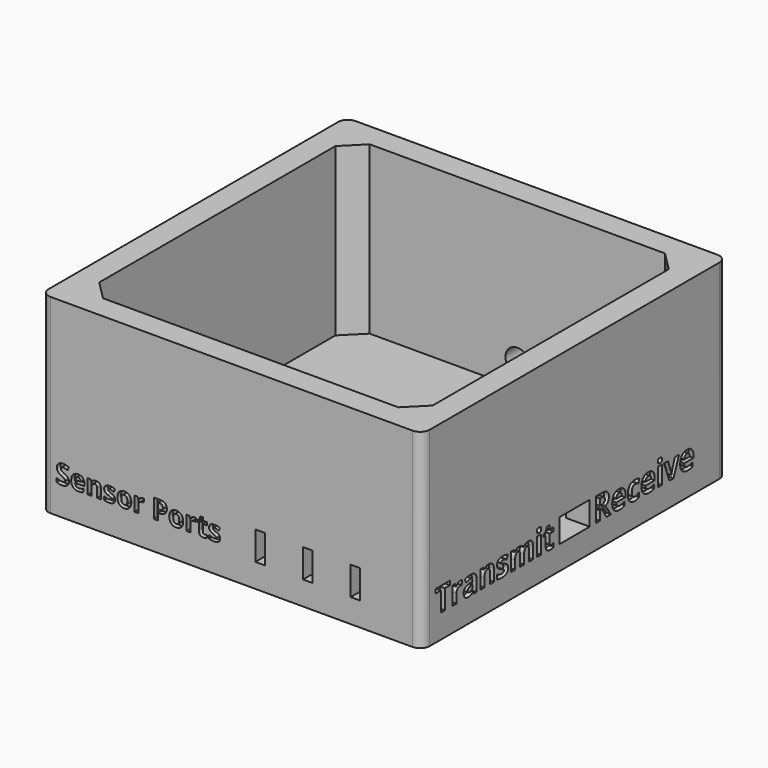
from build123d import *

# Parameters (mm, degrees)
F0_W          = 101.6
F0_H          = 101.6
F1_DEPTH      = 50.8
F2_T          = -6.35
F3_TEXT_SIZE  = 8.8194444444
F4_DEPTH      = 1.27
F5_W          = 10.16
F5_H          = 6.35
F6_DEPTH      = 12.7
F8_R          = 3.175
F9_DEPTH      = 25.4
F7_TEXT_SIZE  = 8.8194444444
F10_DEPTH     = 1.27
F12_DEPTH     = 25.4
F13_TEXT_SIZE = 8.8194444444
F14_DEPTH     = 1.27
F16_TEXT_SIZE = 7.0555555556
F17_DEPTH     = 1.27
F15_W         = 2.54
F15_H         = 7.62
F18_DEPTH     = 25.4
F19_R         = 2.54
F20_SIZE      = 5.08


# Not quite as in the source:
# - Text() gives the source's letters only with a copy of the font that has no kerning and outlines rounded to 1/6400 em; it was checked with that copy


with BuildPart() as f1:
    # F0 (on Top) → F1 (new body)
    with BuildSketch(Plane.XY):
        Rectangle(F0_W, F0_H)
    extrude(amount=F1_DEPTH)

    # F2
    f2_openings = [f1.faces().sort_by_distance(p)[0] for p in [
        (0, 0, 50.8),
    ]]
    offset(amount=F2_T, openings=f2_openings)

    # F3 (on face) → F4 (cut)
    with BuildSketch(Plane.YZ.offset(50.8)):
        with Locations((-46.4357530382, 6.35)):
            Text('Transmit', F3_TEXT_SIZE, font='Open Sans', font_style=FontStyle.BOLD, text_align=(TextAlign.LEFT, TextAlign.BOTTOM))
        with Locations((6.35, 6.35)):
            Text('Receive', F3_TEXT_SIZE, font='Open Sans', font_style=FontStyle.BOLD, text_align=(TextAlign.LEFT, TextAlign.BOTTOM))
    extrude(amount=-F4_DEPTH, mode=Mode.SUBTRACT)

    # F5 (on face) → F6 (cut)
    with BuildSketch(Plane.YZ.offset(50.8)):
        with Locations((0, 9.525)):
            Rectangle(F5_W, F5_H)
    extrude(amount=-F6_DEPTH, mode=Mode.SUBTRACT)

    # F8 (on face) → F9 (cut)
    with BuildSketch(Plane(origin=(0, 50.8, 0), x_dir=(-1, 0, 0), z_dir=(0, 1, 0))):
        with Locations((0, 12.7)):
            Circle(F8_R)
    extrude(amount=-F9_DEPTH, mode=Mode.SUBTRACT)

    # F7 (on face) → F10 (cut)
    with BuildSketch(Plane(origin=(0, 50.8, 0), x_dir=(-1, 0, 0), z_dir=(0, 1, 0))):
        with Locations((-18.8736111111, 18.0932818145)):
            Text('Antenna', F7_TEXT_SIZE, font='Open Sans', font_style=FontStyle.BOLD, text_align=(TextAlign.LEFT, TextAlign.BOTTOM))
    extrude(amount=-F10_DEPTH, mode=Mode.SUBTRACT)

    # F11 (on face) → F12 (cut)
    with BuildSketch(Plane(origin=(-50.8, 0, 0), x_dir=(0, -1, 0), z_dir=(-1, 0, 0))):
        with BuildLine():
            Line((2.54, 11.938), (-2.54, 11.938))
            ThreePointArc((-2.54, 11.938), (-2.9890128061, 11.7520128061), (-3.175, 11.303))
            Line((-3.175, 11.303), (-3.175, 10.795))
            ThreePointArc((-3.175, 10.795), (-2.9890128061, 10.3459871939), (-2.54, 10.16))
            Line((-2.54, 10.16), (2.54, 10.16))
            ThreePointArc((2.54, 10.16), (2.9890128061, 10.3459871939), (3.175, 10.795))
            Line((3.175, 10.795), (3.175, 11.303))
            ThreePointArc((3.175, 11.303), (2.9890128061, 11.7520128061), (2.54, 11.938))
        make_face()
    extrude(amount=-F12_DEPTH, mode=Mode.SUBTRACT)

    # F13 (on face) → F14 (cut)
    with BuildSketch(Plane(origin=(-50.8, 0, 0), x_dir=(0, -1, 0), z_dir=(-1, 0, 0))):
        with Locations((-9.0761299755, 15.24)):
            Text('USB', F13_TEXT_SIZE, font='Open Sans', font_style=FontStyle.BOLD, text_align=(TextAlign.LEFT, TextAlign.BOTTOM))
    extrude(amount=-F14_DEPTH, mode=Mode.SUBTRACT)

    # F16 (on face) → F17 (cut)
    with BuildSketch(Plane.XZ.offset(50.8)):
        with Locations((-46.99, 7.62)):
            Text('Sensor Ports', F16_TEXT_SIZE, font='Open Sans', font_style=FontStyle.BOLD, text_align=(TextAlign.LEFT, TextAlign.BOTTOM))
    extrude(amount=-F17_DEPTH, mode=Mode.SUBTRACT)

    # F15 (on face) → F18 (cut)
    with BuildSketch(Plane.XZ.offset(50.8)):
        with Locations((7.62, 10.16)):
            Rectangle(F15_W, F15_H)
        with Locations((20.32, 10.16)):
            Rectangle(F15_W, F15_H)
        with Locations((33.02, 10.16)):
            Rectangle(F15_W, F15_H)
    extrude(amount=-F18_DEPTH, mode=Mode.SUBTRACT)

    # F19
    f19_edges = [f1.edges().sort_by_distance(p)[0] for p in [
        (-50.8, -50.8, 25.4),
        (50.8, -50.8, 25.4),
        (50.8, 50.8, 25.4),
        (-50.8, 50.8, 25.4),
    ]]
    fillet(f19_edges, radius=F19_R)

    # F20
    f20_edges = [f1.edges().sort_by_distance(p)[0] for p in [
        (-44.45, 44.45, 28.575),
        (44.45, 44.45, 28.575),
        (44.45, -44.45, 28.575),
        (-44.45, -44.45, 28.575),
    ]]
    chamfer(f20_edges, length=F20_SIZE)


solid = f1.part
